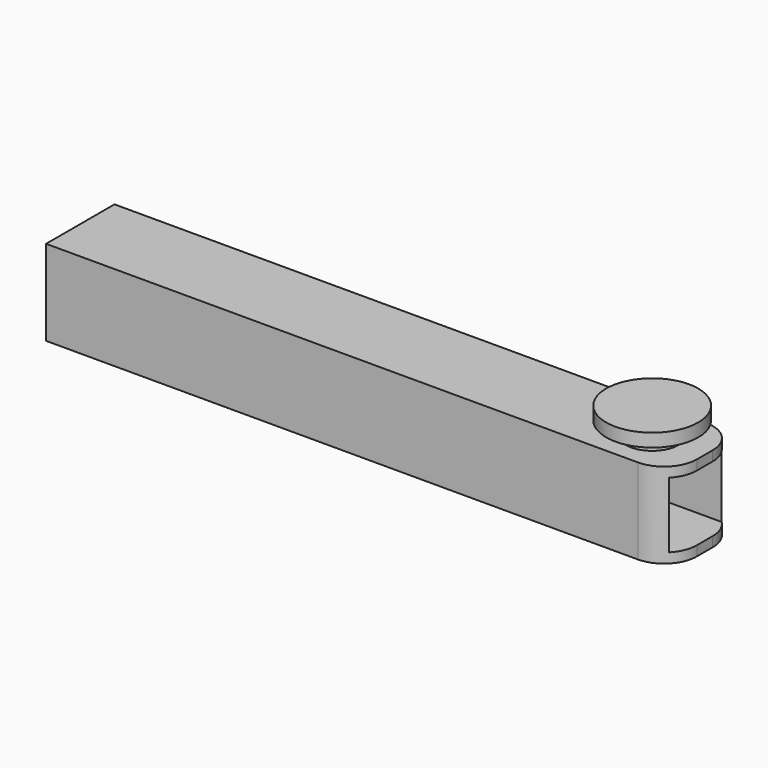
from build123d import *

# Parameters (mm, degrees)
F0_W        = 12.9999973349
F0_H        = 13
F0_W_2      = 10
F0_H_2      = 10
F1_DEPTH    = 95
F2_T1_DEPTH = 38
F3_R        = 4
F4_DEPTH    = 2
F5_R        = 7
F5_R_2      = 4
F6_DEPTH    = 2


# Not quite as in the source:
# - a fillet or chamfer that OpenCascade refuses, or shapes differently, is made with other operations: its cross-section is extruded or revolved along the edge and cut away or added


with BuildPart() as f1:
    # F0 (on Right) → F1 (new body)
    with BuildSketch(Plane.YZ):
        with Locations((-12.2499999048, 6.5)):
            Rectangle(F0_W, F0_H)
        with Locations((-12.2499999048, 6.5)):
            Rectangle(F0_W_2, F0_H_2, mode=Mode.SUBTRACT)
    extrude(amount=F1_DEPTH)

    # F2: fillet of radius 5 on 2 edges, made by hand

    # F2_s2 → F2_t1 (cut)
    with BuildSketch(Plane.XY.offset(-12.5)):
        with BuildLine():
            ThreePointArc((90, -5.7500012374), (93.5355339059, -7.2144673315), (95, -10.7500012374))
            Line((95, -10.7500012374), (95, -5.7500012374))
            Line((95, -5.7500012374), (90, -5.7500012374))
        make_face()
        with BuildLine():
            ThreePointArc((90, -18.7499985722), (93.5355339059, -17.2855324782), (95, -13.7499985722))
            Line((95, -13.7499985722), (95, -18.7499985722))
            Line((95, -18.7499985722), (90, -18.7499985722))
        make_face()
    extrude(amount=F2_T1_DEPTH, mode=Mode.SUBTRACT)

    # F3 (on face) → F4 (join)
    with BuildSketch(Plane.XY.offset(13)):
        with Locations((87, -12.2499999048)):
            Circle(F3_R)
    extrude(amount=F4_DEPTH)

    # F5 (on face) → F6 (join)
    with BuildSketch(Plane.XY.offset(15)):
        with Locations((87, -12.2499999048)):
            Circle(F5_R)
        with Locations((87, -12.2499999048)):
            Circle(F5_R_2, mode=Mode.SUBTRACT)
        with Locations((87, -12.2499999048)):
            Circle(F5_R_2)
    extrude(amount=F6_DEPTH)


solid = f1.part
